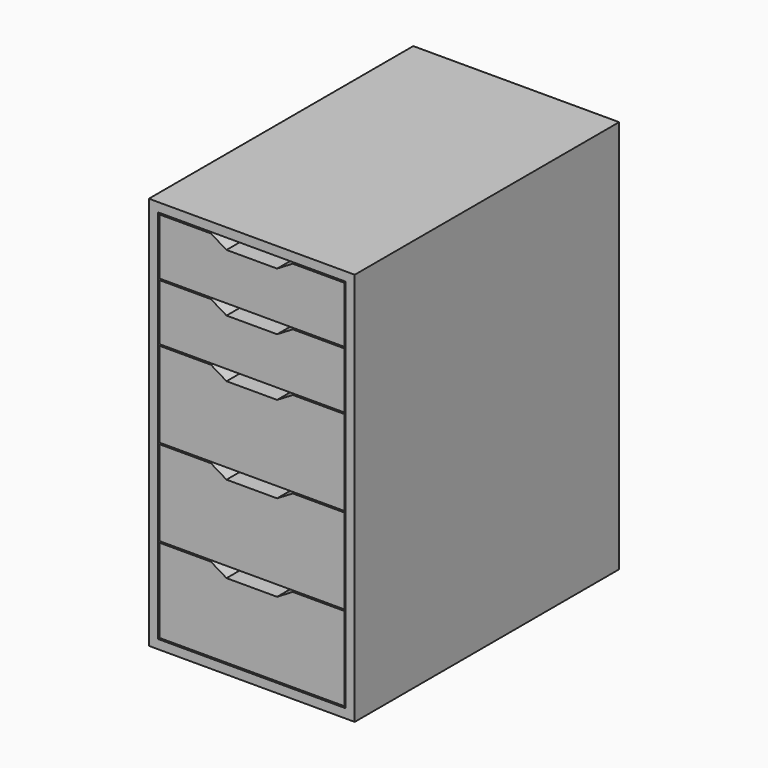
from build123d import *

# Parameters (mm, degrees)
F0_W     = 361.95
F0_H     = 692.15
F1_DEPTH = 581.025
F2_W     = 330.2
F2_H     = 660.4
F3_DEPTH = 565.15
F5_DEPTH = 565.15
F7_DEPTH = 25.4


# Not quite as in the source:
# - a feature names something its author has since deleted; it is built from what else it names


with BuildPart() as f1:
    # F0 (on Front) → F1 (new body)
    with BuildSketch(Plane.XZ):
        with Locations((180.975, 346.075)):
            Rectangle(F0_W, F0_H)
    extrude(amount=F1_DEPTH)

    # F2 (on face) → F3 (cut)
    with BuildSketch(Plane.XZ.offset(581.025)):
        with Locations((180.975, 346.075)):
            Rectangle(F2_W, F2_H)
    extrude(amount=-F3_DEPTH, mode=Mode.SUBTRACT)

    # F4 (on face) → F5 (join)
    with BuildSketch(Plane.XZ.offset(581.025)):
        Polygon((104.775, 168.275), (15.875, 168.275), (15.875, 15.875), (346.075, 15.875), (346.075, 168.275), (257.175, 168.275), (225.425, 149.225), (136.525, 149.225), align=None)
        Polygon((104.775, 676.275), (15.875, 676.275), (15.875, 574.675), (104.775, 574.675), (257.175, 574.675), (346.075, 574.675), (346.075, 676.275), (257.175, 676.275), (225.425, 657.225), (136.525, 657.225), align=None)
        Polygon((104.775, 574.675), (15.875, 574.675), (15.875, 473.075), (104.775, 473.075), (257.175, 473.075), (346.075, 473.075), (346.075, 574.675), (257.175, 574.675), (225.425, 555.625), (136.525, 555.625), align=None)
        Polygon((104.775, 473.075), (15.875, 473.075), (15.875, 320.675), (104.775, 320.675), (257.175, 320.675), (346.075, 320.675), (346.075, 473.075), (257.175, 473.075), (225.425, 454.025), (136.525, 454.025), align=None)
        Polygon((104.775, 320.675), (15.875, 320.675), (15.875, 168.275), (104.775, 168.275), (257.175, 168.275), (346.075, 168.275), (346.075, 320.675), (257.175, 320.675), (225.425, 301.625), (136.525, 301.625), align=None)
    extrude(amount=-F5_DEPTH)

    # F6 (on face) → F7 (cut)
    with BuildSketch(Plane.XZ.offset(581.025)):
        Polygon((257.175, 676.275), (104.775, 676.275), (109.0083333333, 673.735), (252.9416666667, 673.735), align=None)
        Polygon((104.775, 676.275), (15.875, 676.275), (15.875, 15.875), (346.075, 15.875), (346.075, 676.275), (257.175, 676.275), (252.9416666667, 673.735), (343.535, 673.735), (343.535, 574.675), (343.535, 572.135), (343.535, 473.075), (343.535, 470.535), (343.535, 320.675), (343.535, 318.135), (343.535, 168.275), (343.535, 165.735), (343.535, 18.415), (18.415, 18.415), (18.415, 165.735), (18.415, 168.275), (18.415, 318.135), (18.415, 320.675), (18.415, 470.535), (18.415, 473.075), (18.415, 572.135), (18.415, 574.675), (18.415, 673.735), (109.0083333333, 673.735), align=None)
        Polygon((257.175, 574.675), (104.775, 574.675), (109.0083333333, 572.135), (252.9416666667, 572.135), align=None)
        Polygon((104.775, 574.675), (18.415, 574.675), (18.415, 572.135), (109.0083333333, 572.135), align=None)
        Polygon((343.535, 572.135), (343.535, 574.675), (257.175, 574.675), (252.9416666667, 572.135), align=None)
        Polygon((343.535, 470.535), (343.535, 473.075), (257.175, 473.075), (252.9416666667, 470.535), align=None)
        Polygon((257.175, 473.075), (104.775, 473.075), (109.0083333333, 470.535), (252.9416666667, 470.535), align=None)
        Polygon((104.775, 473.075), (18.415, 473.075), (18.415, 470.535), (109.0083333333, 470.535), align=None)
        Polygon((257.175, 320.675), (104.775, 320.675), (109.0083333333, 318.135), (252.9416666667, 318.135), align=None)
        Polygon((104.775, 320.675), (18.415, 320.675), (18.415, 318.135), (109.0083333333, 318.135), align=None)
        Polygon((343.535, 318.135), (343.535, 320.675), (257.175, 320.675), (252.9416666667, 318.135), align=None)
        Polygon((343.535, 165.735), (343.535, 168.275), (257.175, 168.275), (252.9416666667, 165.735), align=None)
        Polygon((108.4452420473, 168.275), (104.775, 168.275), (109.0083333333, 165.735), (252.9416666667, 165.735), (257.175, 168.275), align=None)
        Polygon((104.775, 168.275), (18.415, 168.275), (18.415, 165.735), (109.0083333333, 165.735), align=None)
    extrude(amount=-F7_DEPTH, mode=Mode.SUBTRACT)


solid = f1.part
